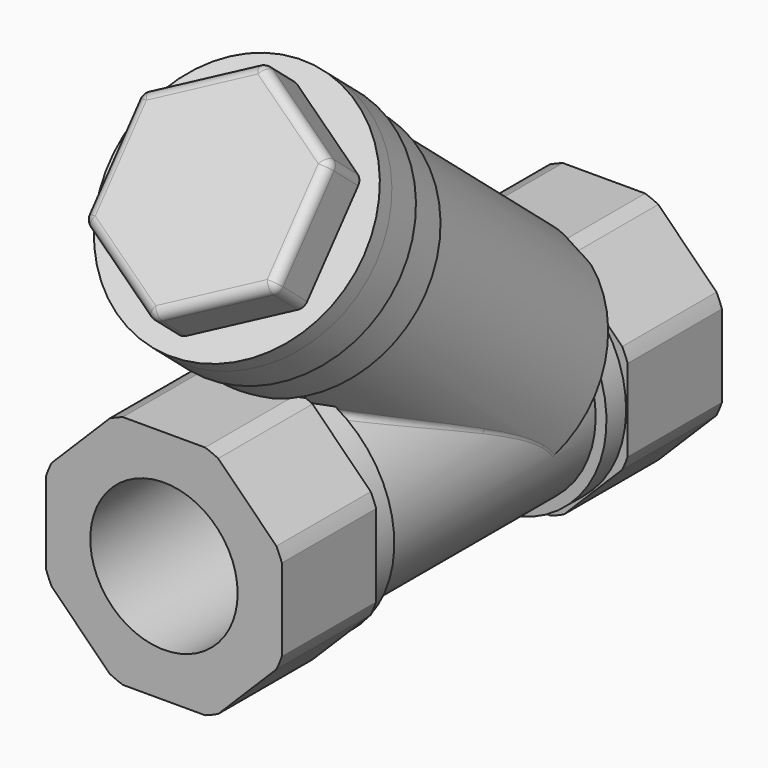
from build123d import *

# Parameters (mm, degrees)
F0_R         = 7.5
F1_DEPTH     = 12
F2_R         = 11.85
F2_R_2       = 7.5
F3_DEPTH     = 2.5
F4_R         = 10.7473655898
F4_R_2       = 7.5
F5_DEPTH     = 13.5
F11_R        = 0.5
F9_FACE_R    = 11.9463172769
F9_FACE_R_2  = 10.9273893647
F12_R        = 12.4463172769
F12_R_2      = 11.9463172769
F13_DEPTH    = 5
F14_R        = 12.9463172769
F14_R_2      = 12.4463172769
F13_FACE_R   = 12.4463172769
F13_FACE_R_2 = 10.9273893647
F15_DEPTH    = 4
F16_R        = 7.5
F17_DEPTH    = 59
F18_R        = 12.9463172769
F19_DEPTH    = 2
F21_DEPTH    = 5
F22_R        = 1


# Not quite as in the source:
# - a feature names something its author has since deleted; it is built from what else it names


with BuildPart() as f1:
    # F0 (on Front) → F1 (new body)
    with BuildSketch(Plane.XZ):
        with BuildLine():
            Line((12, -4.1878177227), (12, 4.1878177227))
            ThreePointArc((12, 4.1878177227), (11.742280513, 4.8638118417), (11.4465156843, 5.5240470642))
            Line((11.4465156843, 5.5240470642), (5.5240470642, 11.4465156843))
            ThreePointArc((5.5240470642, 11.4465156843), (4.8638118417, 11.742280513), (4.1878177227, 12))
            Line((4.1878177227, 12), (-4.1878177227, 12))
            ThreePointArc((-4.1878177227, 12), (-4.8638118417, 11.742280513), (-5.5240470642, 11.4465156843))
            Line((-5.5240470642, 11.4465156843), (-11.4465156843, 5.5240470642))
            ThreePointArc((-11.4465156843, 5.5240470642), (-11.742280513, 4.8638118417), (-12, 4.1878177227))
            Line((-12, 4.1878177227), (-12, -4.1878177227))
            ThreePointArc((-12, -4.1878177227), (-11.742280513, -4.8638118417), (-11.4465156843, -5.5240470642))
            Line((-11.4465156843, -5.5240470642), (-5.5240470642, -11.4465156843))
            ThreePointArc((-5.5240470642, -11.4465156843), (-4.8638118417, -11.742280513), (-4.1878177227, -12))
            Line((-4.1878177227, -12), (4.1878177227, -12))
            ThreePointArc((4.1878177227, -12), (4.8638118417, -11.742280513), (5.5240470642, -11.4465156843))
            Line((5.5240470642, -11.4465156843), (11.4465156843, -5.5240470642))
            ThreePointArc((11.4465156843, -5.5240470642), (11.742280513, -4.8638118417), (12, -4.1878177227))
        make_face()
        Circle(F0_R, mode=Mode.SUBTRACT)
    extrude(amount=F1_DEPTH)

    # F2 (on face) → F3 (join)
    with BuildSketch(Plane.XZ.offset(12)):
        Circle(F2_R)
        Circle(F2_R_2, mode=Mode.SUBTRACT)
    extrude(amount=F3_DEPTH)

    # F4 (on face) → F5 (join)
    with BuildSketch(Plane.XZ.offset(14.5)):
        Circle(F4_R)
        Circle(F4_R_2, mode=Mode.SUBTRACT)
    extrude(amount=F5_DEPTH)

    # F7: F1 across plane


with BuildPart() as f1_1:
    add(f1.part)
    add(f1.part.mirror(Plane.XZ.offset(28)))

    # F8 (on Right) → F9 (revolve)
    with BuildSketch(Plane.YZ):
        Polygon((-24.041232037, -5), (-30, 0), (-45.3208888624, 12.8557521937), (-45.9758430996, 12.0752081286), (-23.9468951734, -6.4092739515), (-16.2679504464, 2.7421360143), (-17.0172415472, 3.3708659006), align=None)
    revolve(axis=Axis((0, -22.0200334247, 7.5687067199), (0, -0.7660444431, 0.6427876097)))

    # F10: union 

    # F11
    f11_edges = [f1_1.edges().sort_by_distance(p)[0] for p in [
        (-10.608197, -23.6012, 1.723957),
        (-8.138636, -34.970086, 7.01915),
        (8.138636, -34.970086, 7.01915),
        (10.608197, -23.6012, 1.723957),
    ]]
    fillet(f11_edges, radius=F11_R)

    # F9_face (on face) + F12 (on face) → F13 (join)
    with BuildSketch(Plane(origin=(0, -38.2968983725, 21.2266180943), x_dir=(1, 0, 0), z_dir=(0, -0.7660444431, 0.6427876097))):
        Circle(F9_FACE_R)
        Circle(F9_FACE_R_2, mode=Mode.SUBTRACT)
    with BuildSketch(Plane(origin=(0, -32.9256115274, 27.6278684889), x_dir=(1, 0, 0), z_dir=(0, -0.7660444431, 0.6427876097))):
        with Locations((0, -8.3562389259)):
            Circle(F12_R)
        with Locations((0, -8.3562389259)):
            Circle(F12_R_2, mode=Mode.SUBTRACT)
    extrude(amount=F13_DEPTH)

    # F14 (on face) + F13_face (on face) → F15 (join)
    with BuildSketch(Plane(origin=(0, -36.755833743, 30.8418065373), x_dir=(1, 0, 0), z_dir=(0, -0.7660444431, 0.6427876097))):
        with Locations((0, -8.3562389259)):
            Circle(F14_R)
        with Locations((0, -8.3562389259)):
            Circle(F14_R_2, mode=Mode.SUBTRACT)
    with BuildSketch(Plane(origin=(0, -42.1271205881, 24.4405561428), x_dir=(1, 0, 0), z_dir=(0, -0.7660444431, 0.6427876097))):
        Circle(F13_FACE_R)
        Circle(F13_FACE_R_2, mode=Mode.SUBTRACT)
    extrude(amount=F15_DEPTH)

    # F16 (on face) → F17 (cut)
    with BuildSketch(Plane.XZ.offset(56)):
        Circle(F16_R)
    extrude(amount=-F17_DEPTH, mode=Mode.SUBTRACT)


with BuildPart() as f19:
    # F18 (on face) → F19 (new body)
    with BuildSketch(Plane(origin=(0, -39.8200115155, 33.4129569761), x_dir=(1, 0, 0), z_dir=(0, -0.7660444431, 0.6427876097))):
        with Locations((0, -8.3562389259)):
            Circle(F18_R)
    extrude(amount=F19_DEPTH)

    # F20 (on face) → F21 (join)
    with BuildSketch(Plane(origin=(0, -41.3521004017, 34.6985321955), x_dir=(1, 0, 0), z_dir=(0, -0.7660444431, 0.6427876097))):
        Polygon((9.75, -2.7270738013), (0, 2.9020913233), (-9.75, -2.7270738013), (-9.75, -13.9854040505), (0, -19.6145691751), (9.75, -13.9854040505), align=None)
    extrude(amount=F21_DEPTH)

    # F22
    f22_edges = [f19.edges().sort_by_distance(p)[0] for p in [
        (0, -41.401783, 38.528632),
        (9.75, -45.020141, 34.216441),
        (9.75, -52.256856, 25.59206),
        (0, -55.875214, 21.279869),
        (-9.75, -52.256856, 25.59206),
        (-9.75, -45.020141, 34.216441),
        (4.875, -55.981146, 25.042934),
        (9.75, -50.553609, 31.51122),
        (4.875, -45.126073, 37.979506),
        (-4.875, -45.126073, 37.979506),
        (-9.75, -50.553609, 31.51122),
        (-4.875, -55.981146, 25.042934),
    ]]
    fillet(f22_edges, radius=F22_R)


solid = Compound([f1_1.part, f19.part])
